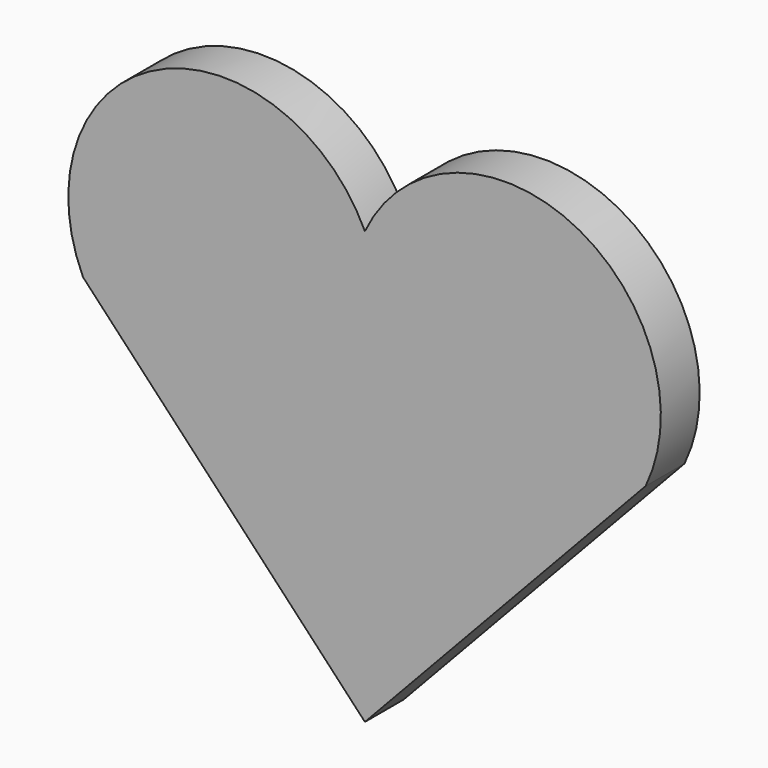
from build123d import *

# Parameters (mm, degrees)
F1_DEPTH = 6.35


with BuildPart() as f1:
    # F0 (on Front) → F1 (new body)
    with BuildSketch(Plane.XZ):
        with BuildLine():
            Line((0, -56.5034113824), (36.7280521826, -17.3911233933))
            ThreePointArc((36.7280521826, -17.3911233933), (27.0872387233, 9.7268599894), (0, 0))
            ThreePointArc((0, 0), (-27.0741003345, 9.7995830277), (-36.8736833622, -17.2745173068))
            Line((-36.8736833622, -17.2745173068), (0, -56.5034113824))
        make_face()
        with BuildLine():
            ThreePointArc((0, -17.2745173068), (-1.9271858798, -8.6372586534), (0, 0))
            ThreePointArc((0, 0), (1.9229070457, -8.6372586534), (0, -17.2745173068))
        make_face(mode=Mode.SUBTRACT)
        with BuildLine():
            ThreePointArc((0, -17.2745173068), (1.9229070457, -8.6372586534), (0, 0))
            ThreePointArc((0, 0), (-1.9271858798, -8.6372586534), (0, -17.2745173068))
        make_face()
    extrude(amount=F1_DEPTH)


solid = f1.part
